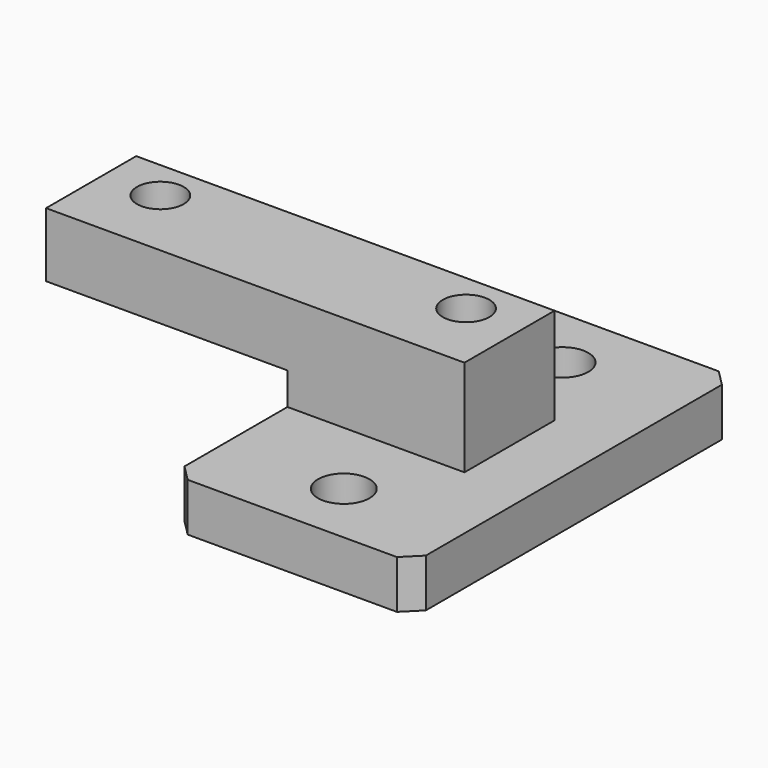
from build123d import *

# Parameters (mm, degrees)
F0_W     = 26
F0_H     = 7
F0_R     = 1.45
F1_DEPTH = 6
F2_W     = 5
F2_H     = 25
F2_R     = 1.6
F3_DEPTH = 3
F4_SIZE  = 1
F6_DEPTH = 2


# Not quite as in the source:
# - a feature of the source that left no trace in its solid (it failed there, or was rolled back) is left out


with BuildPart() as f1:
    # F0 (on Top) → F1 (new body)
    with BuildSketch(Plane.XY):
        with Locations((-13, 3.5)):
            Rectangle(F0_W, F0_H)
        with Locations((-22.5, 4.5)):
            Circle(F0_R, mode=Mode.SUBTRACT)
        with Locations((-3.5, 4.5)):
            Circle(F0_R, mode=Mode.SUBTRACT)
    extrude(amount=F1_DEPTH)

    # F2 (on Top) → F3 (join)
    with BuildSketch(Plane.XY):
        with Locations((1.5, 3.5)):
            Rectangle(F2_W, F2_H)
        with Locations((-3.5, 3.5)):
            Rectangle(F2_W, F2_H)
        with Locations((-3.5, -5)):
            Circle(F2_R, mode=Mode.SUBTRACT)
        with Locations((-3.5, 12)):
            Circle(F2_R, mode=Mode.SUBTRACT)
        with Locations((-8.5, 3.5)):
            Rectangle(F2_W, F2_H)
    extrude(amount=-F3_DEPTH)

    # F4
    f4_edges = [f1.edges().sort_by_distance(p)[0] for p in [
        (4, 16, -1.5),
        (-11, 16, -1.5),
        (4, -9, -1.5),
        (-11, -9, -1.5),
    ]]
    chamfer(f4_edges, length=F4_SIZE)

    # F6 (cut): a face of the model
    f6_faces = [f1.faces().sort_by_distance(p)[0] for p in [
        (-18.2314818077, 3.4328704519, 0),
    ]]
    extrude(f6_faces, amount=-F6_DEPTH, mode=Mode.SUBTRACT)


solid = f1.part
